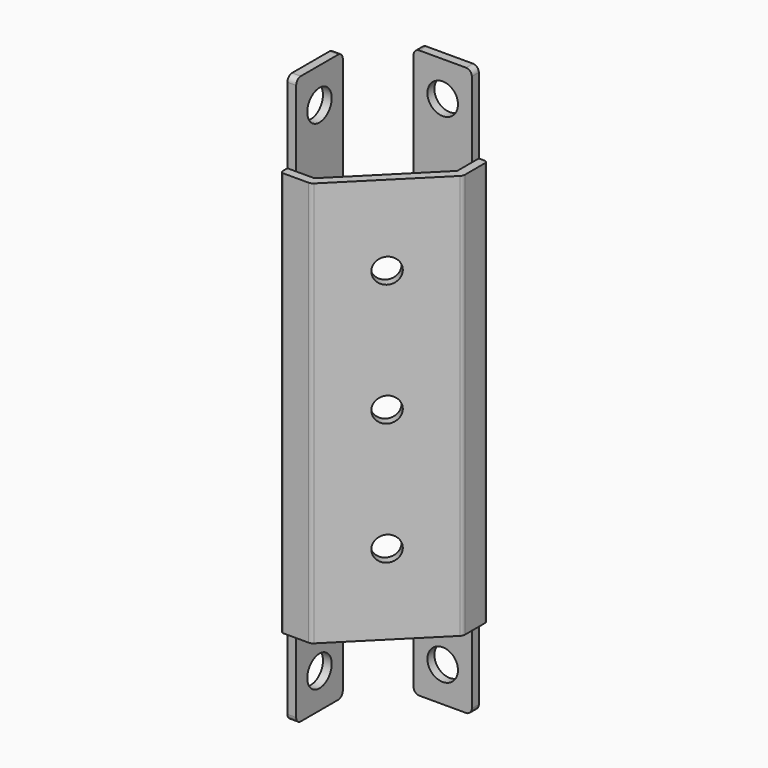
from build123d import *

# Parameters (mm, degrees)
F1_DEPTH = 97.5
F3_DEPTH = 28
F4_R     = 4.25
F5_DEPTH = 25
F6_R     = 5.25
F7_DEPTH = 25
F8_R     = 5.25
F9_DEPTH = 25
F10_R    = 2
F11_R    = 0.5
F12_R    = 1


# Not quite as in the source:
# - a pattern or mirror of a feature is missing from the dataset's text; its kind, count and spacing are read off the source's solid


with BuildPart() as f1:
    # F0 (on Top) → F1 (new body, symmetric)
    with BuildSketch(Plane.XY):
        Polygon((-19.75, 3.25), (-19.75, -19.75), (-9.25, -19.75), (19.75, 9.25), (19.75, 19.75), (-3.25, 19.75), (-3.25, 16.75), (16.75, 16.75), (16.75, 10.4926406871), (-10.4926406871, -16.75), (-16.75, -16.75), (-16.75, 3.25), align=None)
    extrude(amount=F1_DEPTH, both=True)

    # F2 (on face) → F3 (cut)
    with BuildSketch(Plane.XY.offset(97.5)):
        Polygon((-10.4926406871, -16.75), (-16.75, -16.75), (-19.75, -16.75), (-19.75, -19.75), (-9.25, -19.75), (19.75, 9.25), (19.75, 19.75), (16.75, 19.75), (16.75, 16.75), (16.75, 10.4926406871), align=None)
    f3 = extrude(amount=-F3_DEPTH, mode=Mode.SUBTRACT)

    # F3_copies: F3 across plane
    add(f3.mirror(Plane(origin=(0, 0, 0), x_dir=(-1, 0, 0), z_dir=(0, 0, -1))), mode=Mode.SUBTRACT)

    # F4 (on face) → F5 (cut)
    with BuildSketch(Plane(origin=(5.25, -5.25, 0), x_dir=(0.7071067812, 0.7071067812, 0), z_dir=(0.7071067812, -0.7071067812, 0))):
        with Locations((0, 42)):
            Circle(F4_R)
        with Locations((0, -42)):
            Circle(F4_R)
        Circle(F4_R)
    extrude(amount=-F5_DEPTH, mode=Mode.SUBTRACT)

    # F6 (on face) → F7 (cut)
    with BuildSketch(Plane.YZ.offset(-16.75)):
        with Locations((-6.75, 85.5)):
            Circle(F6_R)
        with Locations((-6.75, -85.5)):
            Circle(F6_R)
    extrude(amount=-F7_DEPTH, mode=Mode.SUBTRACT)

    # F8 (on face) → F9 (cut)
    with BuildSketch(Plane.XZ.offset(-16.75)):
        with Locations((6.75, 85.5)):
            Circle(F8_R)
        with Locations((6.75, -85.5)):
            Circle(F8_R)
    extrude(amount=-F9_DEPTH, mode=Mode.SUBTRACT)

    # F10
    f10_edges = [f1.edges().sort_by_distance(p)[0] for p in [
        (-9.25, -19.75, 0),
        (19.75, 9.25, 0),
        (-18.25, -16.75, 97.5),
        (-18.25, 3.25, 97.5),
        (-3.25, 18.25, 97.5),
        (16.75, 18.25, 97.5),
        (-18.25, 3.25, -97.5),
        (-3.25, 18.25, -97.5),
        (-18.25, -16.75, -97.5),
        (16.75, 18.25, -97.5),
    ]]
    fillet(f10_edges, radius=F10_R)

    # F11
    f11_edges = [f1.edges().sort_by_distance(p)[0] for p in [
        (16.75, 10.492641, 0),
        (-10.492641, -16.75, 0),
    ]]
    fillet(f11_edges, radius=F11_R)

    # F12
    f12_edges = [f1.edges().sort_by_distance(p)[0] for p in [
        (-19.75, -19.75, 0),
        (19.75, 19.75, 0),
    ]]
    fillet(f12_edges, radius=F12_R)


solid = f1.part
